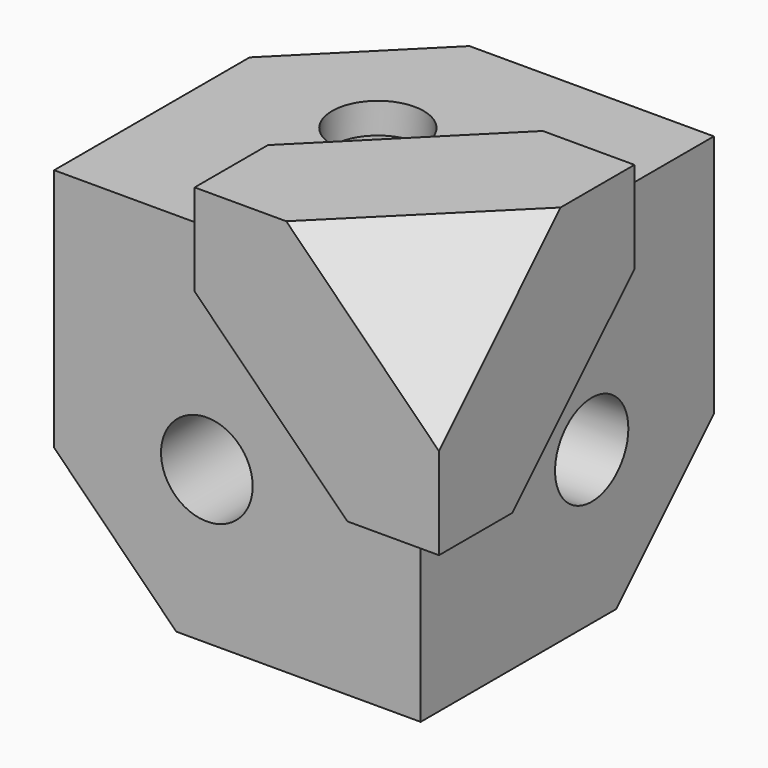
from build123d import *

# Parameters (mm, degrees)
F1_DEPTH     = 3
F0_R         = 1.5
F2_DEPTH     = 2.5
F3_R         = 1.5
F4_DEPTH     = 5.5
F5_DEPTH     = 3
F6_R         = 1.5
F7_DEPTH     = 5.5
F8_DEPTH     = 3
F10_DEPTH    = 5
F11_T4_DEPTH = 32.8926942089
F14_DEPTH    = 0.3
F15_R        = 0.29999
F16_R        = 1
F17_R        = 0.2
F18_DEPTH    = 1
F19_DEPTH    = 1
F20_DEPTH    = 1
F21_R        = 1.5
F22_DEPTH    = 2.5
F23_DEPTH    = 1
F24_DEPTH    = 0.05
F26_DEPTH    = 0.6
F27_SIZE     = 0.3


# Not quite as in the source:
# - a fillet or chamfer that OpenCascade refuses, or shapes differently, is made with other operations: its cross-section is extruded or revolved along the edge and cut away or added
# - a fillet or chamfer is up to 0.001 mm smaller than in the source, because OpenCascade refuses the exact size


with BuildPart() as f1:
    # F0 (on Front) → F1 (new body)
    with BuildSketch(Plane.XZ):
        Polygon((15.2273818341, 37.2200216049), (7.2273818341, 37.2200216049), (7.2273818341, 34.2200216049), (12.2273818341, 29.2200216049), (15.2273818341, 29.2200216049), align=None)
    extrude(amount=F1_DEPTH)

    # F0 (on Front) → F2 (join)
    with BuildSketch(Plane.XZ):
        Polygon((7.2273818341, 34.2200216049), (7.2273818341, 37.2200216049), (0.2273818341, 37.2200216049), (0.2273818341, 26.2200216049), (4.2273818341, 22.2200216049), (15.2273818341, 22.2200216049), (15.2273818341, 29.2200216049), (12.2273818341, 29.2200216049), align=None)
        with Locations((5.2273818341, 27.2200216049)):
            Circle(F0_R, mode=Mode.SUBTRACT)
        Polygon((15.2273818341, 37.2200216049), (7.2273818341, 37.2200216049), (7.2273818341, 34.2200216049), (12.2273818341, 29.2200216049), (15.2273818341, 29.2200216049), align=None)
    extrude(amount=-F2_DEPTH)

    # F3 (on face) → F4 (join)
    with BuildSketch(Plane.XY.offset(37.2200216049)):
        Polygon((0.2273818341, 2.5), (9.7273818341, 2.5), (12.2273818341, 5), (12.2273818341, 12), (4.2273818341, 12), (0.2273818341, 8), align=None)
        with Locations((5.2273818341, 7)):
            Circle(F3_R, mode=Mode.SUBTRACT)
        Polygon((9.7273818341, 2.5), (15.2273818341, 2.5), (15.2273818341, 5), (12.2273818341, 5), align=None)
    extrude(amount=-F4_DEPTH)

    # F3 (on face) → F5 (cut)
    with BuildSketch(Plane.XY.offset(37.2200216049)):
        Polygon((0.2273818341, 2.5), (9.7273818341, 2.5), (12.2273818341, 5), (12.2273818341, 12), (4.2273818341, 12), (0.2273818341, 8), align=None)
        with Locations((5.2273818341, 7)):
            Circle(F3_R, mode=Mode.SUBTRACT)
        Polygon((0.2273818341, 0), (7.2273818341, 0), (9.7273818341, 2.5), (0.2273818341, 2.5), align=None)
    extrude(amount=-F5_DEPTH, mode=Mode.SUBTRACT)

    # F6 (on face) → F7 (join)
    with BuildSketch(Plane.YZ.offset(15.2273818341)):
        Polygon((5, 34.2200216049), (0, 29.2200216049), (0, 22.2200216049), (8, 22.2200216049), (12, 26.2200216049), (12, 34.2200216049), align=None)
        with Locations((7, 27.2200216049)):
            Circle(F6_R, mode=Mode.SUBTRACT)
    extrude(amount=-F7_DEPTH)

    # F6 (on face) → F8 (cut)
    with BuildSketch(Plane.YZ.offset(15.2273818341)):
        Polygon((2.5, 31.7200216049), (0, 29.2200216049), (0, 22.2200216049), (2.5, 22.2200216049), align=None)
        Polygon((5, 31.7200216049), (2.5, 31.7200216049), (2.5, 22.2200216049), (8, 22.2200216049), (12, 26.2200216049), (12, 34.2200216049), (5, 34.2200216049), align=None)
        with Locations((7, 27.2200216049)):
            Circle(F6_R, mode=Mode.SUBTRACT)
        Polygon((5, 34.2200216049), (2.5, 31.7200216049), (5, 31.7200216049), align=None)
    extrude(amount=-F8_DEPTH, mode=Mode.SUBTRACT)

    # F9 (on face) → F10 (cut)
    with BuildSketch(Plane.XZ.offset(3)):
        Polygon((15.2273818341, 32.2200216049), (15.2273818341, 37.2200216049), (10.2273818341, 37.2200216049), align=None)
    extrude(amount=-F10_DEPTH, mode=Mode.SUBTRACT)

    # F11: chamfer of 5 x 3.5533150469 on 1 edges, made by hand


with BuildPart() as f11_tool2:
    # F11_s3 → F11_t4 (new body)
    with BuildSketch(Plane(origin=(-22.6256434487, 0, 22.6256434487), x_dir=(0, 1, 0), z_dir=(0.7071067812, 0, -0.7071067812))):
        Polygon((2, 37.1036957683), (-3, 33.5503807214), (2, 33.5503807214), align=None)
    extrude(amount=F11_T4_DEPTH)

    split(bisect_by=Plane.YZ.offset(15.2273818341), keep=Keep.BOTTOM)

    split(bisect_by=Plane.XZ.offset(3), keep=Keep.BOTTOM)

    split(bisect_by=Plane.XY.offset(37.2200216049), keep=Keep.BOTTOM)


with BuildPart() as f1_1:
    add(f1.part)

    # F11_t1: union F11_tool2
    add(f11_tool2.part)

    # F13 (on 3pt) → F14 (cut, symmetric)
    with BuildSketch(Plane(origin=(13.8158011463, -13.8158011463, 13.8158011463), x_dir=(0.8164965809, 0.4082482905, -0.4082482905), z_dir=(0.5773502692, -0.5773502692, 0.5773502692))):
        Polygon((-1.0654091424, 19.1374719877), (-1.0654091424, 29.2569466706), (-9.8291312908, 24.1972093292), align=None)
        Polygon((-1.9454084062, 20.6616754232), (-8.0691327632, 24.1972093292), (-1.9454084062, 27.7327432351), align=None, mode=Mode.SUBTRACT)
        Polygon((-1.9454084062, 27.7327432351), (-8.0691327632, 24.1972093292), (-1.9454084062, 20.6616754232), align=None)
        Polygon((-7.6691327632, 24.1972093292), (-2.1454084062, 27.3863330736), (-2.1454084062, 21.0080855847), align=None, mode=Mode.SUBTRACT)
    extrude(amount=F14_DEPTH, both=True, mode=Mode.SUBTRACT)

    # F15 (radius 0.3 in the source; OpenCascade refuses exactly that, so slightly less here)
    f15_edges = [f1_1.edges().sort_by_distance(p)[0] for p in [
        (9.635826, 2.591555, 33.883517),
        (11.890877, 2.591555, 31.628466),
        (9.982237, 2.245145, 34.229927),
        (12.237288, 2.245145, 31.974876),
        (9.635826, 0.336504, 31.628466),
        (9.982237, -0.009906, 31.974876),
    ]]
    fillet(f15_edges, radius=F15_R)

    # F16
    f16_edges = [f1_1.edges().sort_by_distance(p)[0] for p in [
        (12.746997, 2.5, 31.720022),
        (9.727382, -0.519615, 31.720022),
        (9.727382, 2.5, 34.739637),
    ]]
    fillet(f16_edges, radius=F16_R)

    # F17
    f17_edges = [f1_1.edges().sort_by_distance(p)[0] for p in [
        (9.467574, 0, 31.460214),
        (12.227382, 2.759808, 31.460214),
        (9.467574, 2.759808, 34.220022),
    ]]
    fillet(f17_edges, radius=F17_R)

    # F18 (add): a face of the model
    f18_faces = [f1_1.faces().sort_by_distance(p)[0] for p in [
        (4.9773818341, 2.5, 31.5856713165),
    ]]
    extrude(f18_faces, amount=F18_DEPTH)

    # F19 (add): a face of the model
    f19_faces = [f1_1.faces().sort_by_distance(p)[0] for p in [
        (9.7273818341, 7.75, 31.592546117),
    ]]
    extrude(f19_faces, amount=F19_DEPTH)

    # F20 (add): a face of the model
    f20_faces = [f1_1.faces().sort_by_distance(p)[0] for p in [
        (4.4773818341, 3.6202081528, 31.7200216049),
    ]]
    extrude(f20_faces, amount=F20_DEPTH)

    # F21 (on face) → F22 (cut)
    with BuildSketch(Plane(origin=(0, 0, 30.7200216049), x_dir=(1, 0, 0), z_dir=(0, 0, -1))):
        Polygon((2.0765037567, -7.8442752363), (4.3831065978, -10.1508780774), (5.0592546763, -9.9697047458), (4.9816089627, -9.679926998), (6.7801908833, -9.1979984248), (6.8578365969, -9.4877761727), (7.5339846753, -9.3066028411), (8.3782599116, -6.1557247637), (6.0716570704, -3.8491219226), (2.920778993, -4.6933971589), (2.7396056614, -5.3695452373), (3.0293834093, -5.4471909508), (2.5474548362, -7.2457728714), (2.2576770883, -7.1681271579), align=None)
        with Locations((5.2273818341, -7)):
            Circle(F21_R, mode=Mode.SUBTRACT)
        Polygon((2.7396056614, -5.3695452373), (2.2576770883, -7.1681271579), (2.5474548362, -7.2457728714), (3.0293834093, -5.4471909508), align=None)
        Polygon((4.9816089627, -9.679926998), (5.0592546763, -9.9697047458), (6.8578365969, -9.4877761727), (6.7801908833, -9.1979984248), align=None)
    extrude(amount=-F22_DEPTH, mode=Mode.SUBTRACT)

    # F21 (on face) → F23 (cut)
    with BuildSketch(Plane(origin=(0, 0, 30.7200216049), x_dir=(1, 0, 0), z_dir=(0, 0, -1))):
        Polygon((0.7242075999, -7.4819285731), (2.0765037567, -7.8442752363), (2.2576770883, -7.1681271579), (1.5815290099, -6.9869538263), (2.063457583, -5.1883719057), (2.7396056614, -5.3695452373), (2.920778993, -4.6933971589), (1.5684828362, -4.3310504957), align=None)
        Polygon((5.0592546763, -9.9697047458), (4.3831065978, -10.1508780774), (4.745453261, -11.5031742342), (7.8963313384, -10.6588989979), (7.5339846753, -9.3066028411), (6.8578365969, -9.4877761727), (7.0390099284, -10.1639242511), (5.2404280078, -10.6458528242), align=None)
    extrude(amount=-F23_DEPTH, mode=Mode.SUBTRACT)

    # F21 (on face) → F24 (join, symmetric)
    with BuildSketch(Plane(origin=(0, 0, 30.7200216049), x_dir=(1, 0, 0), z_dir=(0, 0, -1))):
        Polygon((1.5815290099, -6.9869538263), (2.2576770883, -7.1681271579), (2.7396056614, -5.3695452373), (2.063457583, -5.1883719057), align=None)
        Polygon((6.8578365969, -9.4877761727), (5.0592546763, -9.9697047458), (5.2404280078, -10.6458528242), (7.0390099284, -10.1639242511), align=None)
    extrude(amount=F24_DEPTH, both=True)

    # F25 (on face) → F26 (join)
    with BuildSketch(Plane(origin=(0, 0, 30.6700216049), x_dir=(1, 0, 0), z_dir=(0, 0, -1))):
        Polygon((2.7396056614, -5.3695452373), (2.2576770883, -7.1681271579), (2.7406400014, -7.2975366804), (3.2225685746, -5.4989547598), align=None)
        Polygon((1.5815290099, -6.9869538263), (2.2576770883, -7.1681271579), (2.7396056614, -5.3695452373), (2.063457583, -5.1883719057), align=None)
        Polygon((4.9298451537, -9.4867418327), (5.0592546763, -9.9697047458), (6.8578365969, -9.4877761727), (6.7284270743, -9.0048132595), align=None)
        Polygon((5.0592546763, -9.9697047458), (5.2404280078, -10.6458528242), (7.0390099284, -10.1639242511), (6.8578365969, -9.4877761727), align=None)
    extrude(amount=F26_DEPTH)

    # F27
    f27_edges = [f1_1.edges().sort_by_distance(p)[0] for p in [
        (2.981604, 6.398246, 30.070022),
        (5.829136, 9.245778, 30.070022),
    ]]
    chamfer(f27_edges, length=F27_SIZE)


solid = f1_1.part
